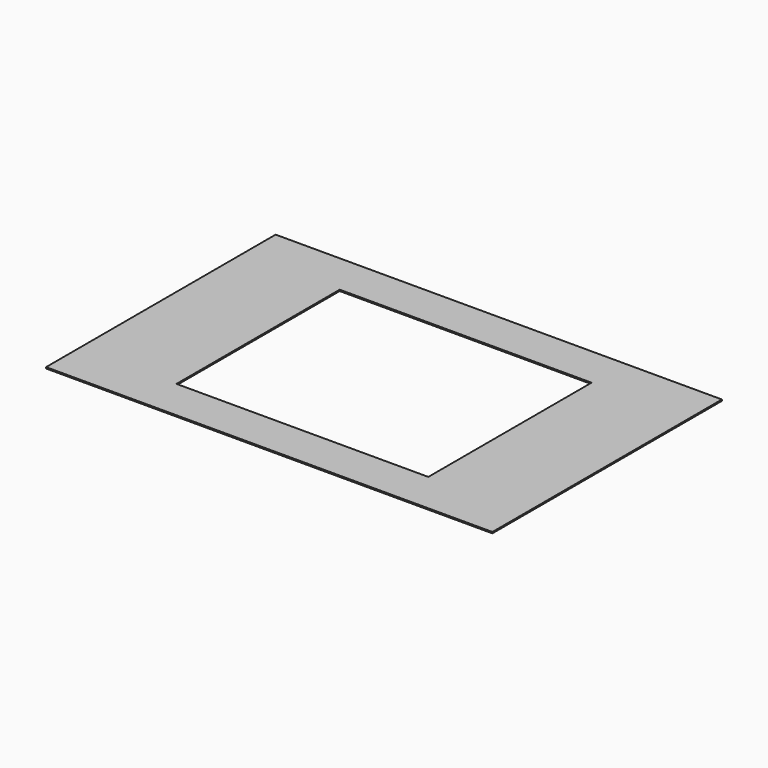
from build123d import *

# Parameters (mm, degrees)
F2_DEPTH = 2


# Not quite as in the source:
# - the program builds the solid bodies; features that only make, move or delete a surface that nothing else refers to are left out


with BuildPart() as f2:
    # F0 (on Top) → F2 (new body)
    with BuildSketch(Plane.XY):
        Polygon((-350, -225), (350, -225), (350, -217.2532975674), (350, 225), (-350, 225), align=None)
        with BuildLine():
            Line((197.5, 160), (197.5, -160))
            Line((197.5, -160), (-197.5, -160))
            Line((-197.5, -160), (-197.5, 84.3677148223))
            Line((-197.5, 84.3677148223), (-197.5, 160))
            Line((-197.5, 160), (-84.6111023318, 160))
            ThreePointArc((-84.6111023318, 160), (-82.6551501399, 160.0153039327), (-80.699197948, 160))
            Line((-80.699197948, 160), (197.5, 160))
        make_face(mode=Mode.SUBTRACT)
    extrude(amount=F2_DEPTH)


solid = f2.part
